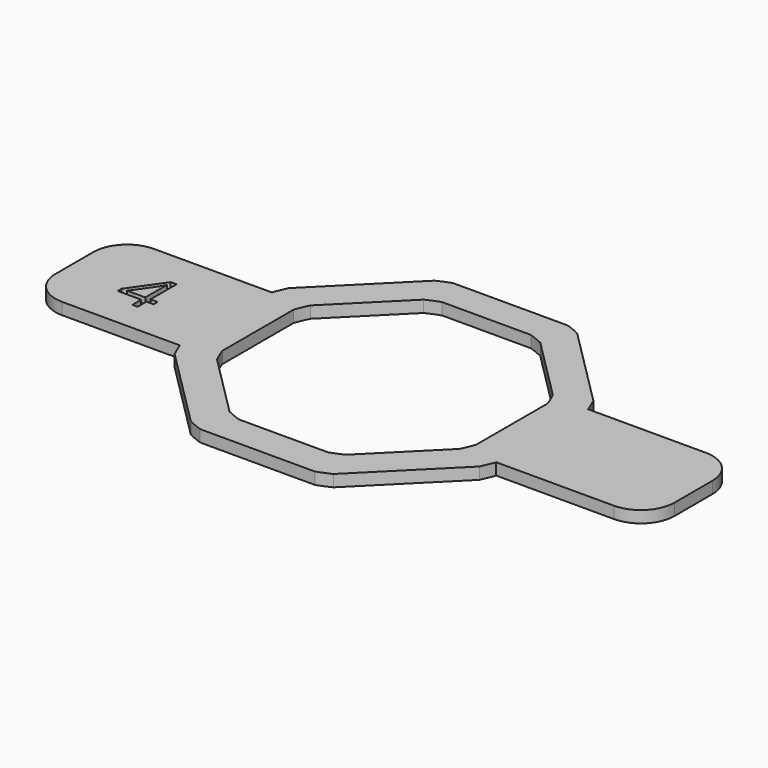
from build123d import *

# Parameters (mm, degrees)
F1_DEPTH     = 1.27
F2_DEPTH     = 1.27
F3_DEPTH     = 1.27
F0_TEXT_SIZE = 7.316316866
F4_DEPTH     = 0.635


# Not quite as in the source:
# - Text() gives the source's letters only with a copy of the font that has no kerning and outlines rounded to 1/6400 em; it was checked with that copy


with BuildPart() as f1:
    # F0 (on Top) → F1 (new body)
    with BuildSketch(Plane.XY):
        with BuildLine():
            Line((-7.6822955443, 16.4361066094), (-16.4361066094, 7.6822955443))
            ThreePointArc((-16.4361066094, 7.6822955443), (-16.7618143756, 6.9429708443), (-17.0542857143, 6.1898791653))
            Line((-17.0542857143, 6.1898791653), (-17.0542857143, -6.1898791653))
            ThreePointArc((-17.0542857143, -6.1898791653), (-16.7618143756, -6.9429708443), (-16.4361066094, -7.6822955443))
            Line((-16.4361066094, -7.6822955443), (-7.6822955443, -16.4361066094))
            ThreePointArc((-7.6822955443, -16.4361066094), (-6.9429708443, -16.7618143756), (-6.1898791653, -17.0542857143))
            Line((-6.1898791653, -17.0542857143), (6.1898791653, -17.0542857143))
            ThreePointArc((6.1898791653, -17.0542857143), (6.9429708443, -16.7618143756), (7.6822955443, -16.4361066094))
            Line((7.6822955443, -16.4361066094), (16.4361066094, -7.6822955443))
            ThreePointArc((16.4361066094, -7.6822955443), (16.7618143756, -6.9429708443), (17.0542857143, -6.1898791653))
            Line((17.0542857143, -6.1898791653), (17.0542857143, 6.1898791653))
            ThreePointArc((17.0542857143, 6.1898791653), (16.7618143756, 6.9429708443), (16.4361066094, 7.6822955443))
            Line((16.4361066094, 7.6822955443), (7.6822955443, 16.4361066094))
            ThreePointArc((7.6822955443, 16.4361066094), (6.9429708443, 16.7618143756), (6.1898791653, 17.0542857143))
            Line((6.1898791653, 17.0542857143), (-6.1898791653, 17.0542857143))
            ThreePointArc((-6.1898791653, 17.0542857143), (-6.9429708443, 16.7618143756), (-7.6822955443, 16.4361066094))
        make_face()
        with BuildLine():
            ThreePointArc((13.1226804028, 6.3623217967), (13.452672622, 5.6244624066), (13.7410782644, 4.8693772923))
            Line((13.7410782644, 4.8693772923), (13.7410782644, -4.7292058301))
            ThreePointArc((13.7410782644, -4.7292058301), (13.452672622, -5.4842909444), (13.1226804028, -6.2221503345))
            Line((13.1226804028, -6.2221503345), (6.3354571871, -13.0093735502))
            ThreePointArc((6.3354571871, -13.0093735502), (5.597597797, -13.3393657694), (4.8425126828, -13.6277714118))
            Line((4.8425126828, -13.6277714118), (-4.7560704397, -13.6277714118))
            ThreePointArc((-4.7560704397, -13.6277714118), (-5.5111555539, -13.3393657694), (-6.249014944, -13.0093735502))
            Line((-6.249014944, -13.0093735502), (-13.0362381597, -6.2221503345))
            ThreePointArc((-13.0362381597, -6.2221503345), (-13.3662303789, -5.4842909444), (-13.6546360213, -4.7292058301))
            Line((-13.6546360213, -4.7292058301), (-13.6546360213, 4.8693772923))
            ThreePointArc((-13.6546360213, 4.8693772923), (-13.3662303789, 5.6244624066), (-13.0362381597, 6.3623217967))
            Line((-13.0362381597, 6.3623217967), (-6.249014944, 13.1495450124))
            ThreePointArc((-6.249014944, 13.1495450124), (-5.5111555539, 13.4795372315), (-4.7560704397, 13.767942874))
            Line((-4.7560704397, 13.767942874), (4.8425126828, 13.767942874))
            ThreePointArc((4.8425126828, 13.767942874), (5.597597797, 13.4795372315), (6.3354571871, 13.1495450124))
            Line((6.3354571871, 13.1495450124), (13.1226804028, 6.3623217967))
        make_face(mode=Mode.SUBTRACT)
    extrude(amount=F1_DEPTH)

    # F0 (on Top) → F2 (join)
    with BuildSketch(Plane.XY):
        with BuildLine():
            Line((-17.0542857143, -6.1898791653), (-17.0542857143, 6.1898791653))
            Line((-17.0542857143, 6.1898791653), (-29.7542857143, 6.1898791653))
            ThreePointArc((-29.7542857143, 6.1898791653), (-32.3200731774, 5.1270951999), (-33.3828571429, 2.5613077368))
            Line((-33.3828571429, 2.5613077368), (-33.3828571429, -2.5613077368))
            ThreePointArc((-33.3828571429, -2.5613077368), (-32.3200731774, -5.1270951999), (-29.7542857143, -6.1898791653))
            Line((-29.7542857143, -6.1898791653), (-17.0542857143, -6.1898791653))
        make_face()
        Polygon((-23.4643447247, -1.1766624078), (-23.4643447247, -1.7162407767), (-24.2394170427, -1.7162407767), (-24.2394170427, -2.9165740125), (-24.8075747744, -2.9165740125), (-24.8075747744, -1.7162407767), (-27.3477085363, -1.7162407767), (-27.3477085363, -1.1983827235), (-24.8681630234, 2.3351696879), (-24.2394170427, 2.3351696879), (-24.2394170427, -1.1766624078), align=None, mode=Mode.SUBTRACT)
        with BuildLine():
            Line((29.7542857143, 6.1898791653), (17.0542857143, 6.1898791653))
            Line((17.0542857143, 6.1898791653), (17.0542857143, -6.1898791653))
            Line((17.0542857143, -6.1898791653), (29.7542857143, -6.1898791653))
            ThreePointArc((29.7542857143, -6.1898791653), (32.3200731774, -5.1270951999), (33.3828571429, -2.5613077368))
            Line((33.3828571429, -2.5613077368), (33.3828571429, 2.5613077368))
            ThreePointArc((33.3828571429, 2.5613077368), (32.3200731774, 5.1270951999), (29.7542857143, 6.1898791653))
        make_face()
    extrude(amount=F2_DEPTH)


with BuildPart() as f3:
    # F0 (on Top) → F3 (new body)
    with BuildSketch(Plane.XY):
        with BuildLine():
            Line((-26.7544009654, -1.1766624078), (-24.8075747744, -1.1766624078))
            Line((-24.8075747744, -1.1766624078), (-24.8075747744, 0.5598196734))
            add(Edge.make_bspline(
                [(-24.8075747744, 0.5598196734), (-24.8075747744, 1.0708186795), (-24.77099319, 1.7132827543)],
                knots=[0, 0, 0, 1, 1, 1], degree=2))
            Line((-24.77099319, 1.7132827543), (-24.7995725528, 1.7132827543))
            add(Edge.make_bspline(
                [(-24.7995725528, 1.7132827543), (-24.9710487293, 1.3703304012), (-25.1219477647, 1.1451250227)],
                knots=[0, 0, 0, 1, 1, 1], degree=2))
            Line((-25.1219477647, 1.1451250227), (-26.7544009654, -1.1766624078))
        make_face()
    extrude(amount=F3_DEPTH)


with BuildPart() as f4:
    # F0 (on Top) → F4 (new body)
    with BuildSketch(Plane.XY):
        with Locations((-27.5008939207, -2.9165740125)):
            Text('4', F0_TEXT_SIZE, font='Open Sans', text_align=(TextAlign.LEFT, TextAlign.BOTTOM))
    extrude(amount=F4_DEPTH)


solid = Compound([f1.part, f3.part, f4.part])
